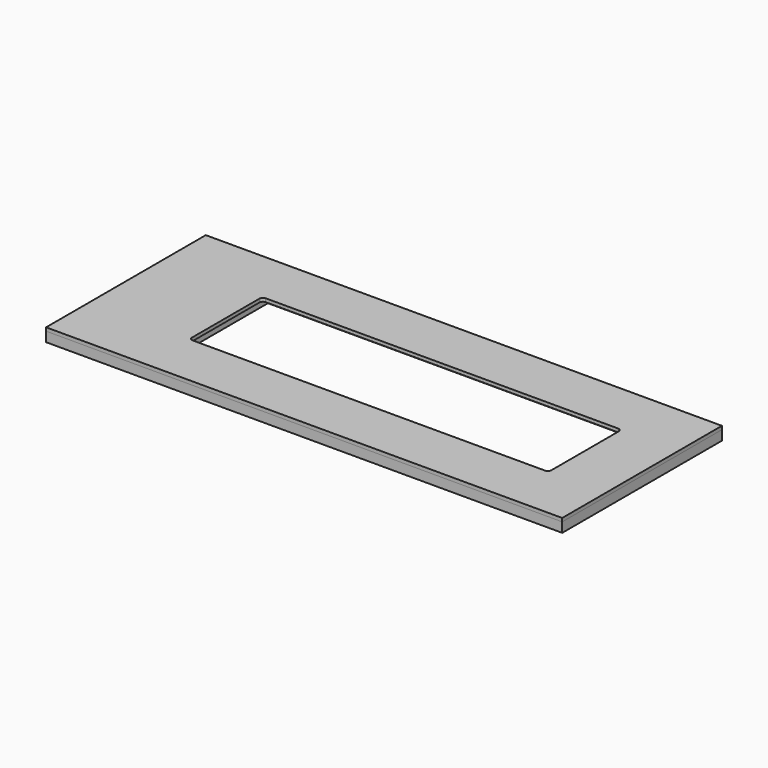
from build123d import *

# Parameters (mm, degrees)
F0_W     = 905
F0_H     = 350
F1_DEPTH = 6
F2_W     = 60
F2_H     = 210
F2_W_2   = 70
F3_DEPTH = 17


# Not quite as in the source:
# - a feature of the source that left no trace in its solid (it failed there, or was rolled back) is left out


with BuildPart() as f1:
    # F0 (on Top) → F1 (new body)
    with BuildSketch(Plane.XY):
        Rectangle(F0_W, F0_H)
        with BuildLine():
            ThreePointArc((-277.5, 74), (-275.7426406871, 78.2426406871), (-271.5, 80))
            Line((-271.5, 80), (346.5, 80))
            ThreePointArc((346.5, 80), (350.7426406871, 78.2426406871), (352.5, 74))
            Line((352.5, 74), (352.5, -74))
            ThreePointArc((352.5, -74), (350.7426406871, -78.2426406871), (346.5, -80))
            Line((346.5, -80), (-271.5, -80))
            ThreePointArc((-271.5, -80), (-275.7426406871, -78.2426406871), (-277.5, -74))
            Line((-277.5, -74), (-277.5, 74))
        make_face(mode=Mode.SUBTRACT)
    extrude(amount=F1_DEPTH)


with BuildPart() as f3:
    # F2 (on face) → F3 (new body)
    with BuildSketch(Plane(origin=(0, 0, 0), x_dir=(1, 0, 0), z_dir=(0, 0, -1))):
        with Locations((422.5, 0)):
            Rectangle(F2_W, F2_H)
        Polygon((452.5, 175), (-452.5, 175), (-452.5, 105), (-357.5, 105), (-287.5, 105), (392.5, 105), (452.5, 105), align=None)
        Polygon((-357.5, -105), (-452.5, -105), (-452.5, -175), (452.5, -175), (452.5, -105), (392.5, -105), (-287.5, -105), align=None)
        with Locations((-322.5, 0)):
            Rectangle(F2_W_2, F2_H)
    extrude(amount=F3_DEPTH)


solid = Compound([f1.part, f3.part])
